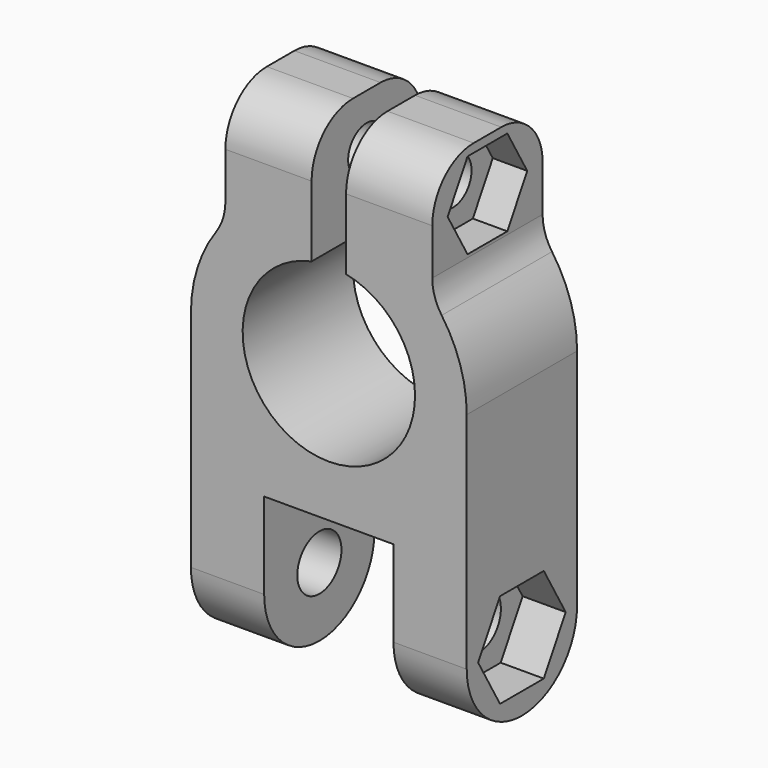
from build123d import *

# Parameters (mm, degrees)
F1_DEPTH = 4
F2_R     = 1.35
F3_DEPTH = 14.001
F4_DEPTH = 2
F5_R     = 1.6
F6_DEPTH = 25
F7_DEPTH = 2.5
F8_SIZE  = 1.35
F9_R     = 3
F10_R    = 3.99999
F11_SIZE = 1.55


# Not quite as in the source:
# - a fillet or chamfer is up to 0.001 mm smaller than in the source, because OpenCascade refuses the exact size
# - a feature names something its author has since deleted; it is built from what else it names


with BuildPart() as f1:
    # F0 (on Front) → F1 (new body, symmetric)
    with BuildSketch(Plane.XZ):
        with BuildLine():
            ThreePointArc((1, 4.8989794856), (0, -5), (-1, 4.8989794856))
            Line((-1, 4.8989794856), (-1, 12))
            Line((-1, 12), (-6, 12))
            Line((-6, 12), (-6, 5.2915026221))
            ThreePointArc((-6, 5.2915026221), (-7.4833147735, 2.8284271247), (-8, 0))
            Line((-8, 0), (-8, -17))
            Line((-8, -17), (-3.75, -17))
            Line((-3.75, -17), (-3.75, -8))
            Line((-3.75, -8), (3.75, -8))
            Line((3.75, -8), (3.75, -17))
            Line((3.75, -17), (8, -17))
            Line((8, -17), (8, 0))
            ThreePointArc((8, 0), (7.4833147735, 2.8284271247), (6, 5.2915026221))
            Line((6, 5.2915026221), (6, 12))
            Line((6, 12), (1, 12))
            Line((1, 12), (1, 4.8989794856))
        make_face()
    extrude(amount=F1_DEPTH, both=True)

    # F2 (on face) → F3 (cut, through all)
    with BuildSketch(Plane.YZ.offset(6)):
        with Locations((0, 9)):
            Circle(F2_R)
    extrude(amount=-F3_DEPTH, mode=Mode.SUBTRACT)

    # F2 (on face) → F4 (cut)
    with BuildSketch(Plane.YZ.offset(6)):
        Polygon((2.8867513459, 9), (1.443375673, 11.5), (-1.443375673, 11.5), (-2.8867513459, 9), (-1.443375673, 6.5), (1.443375673, 6.5), align=None)
        with Locations((0, 9)):
            Circle(F2_R, mode=Mode.SUBTRACT)
    extrude(amount=-F4_DEPTH, mode=Mode.SUBTRACT)

    # F5 (on face) → F6 (cut)
    with BuildSketch(Plane.YZ.offset(8)):
        with Locations((0, -13)):
            Circle(F5_R)
    extrude(amount=-F6_DEPTH, mode=Mode.SUBTRACT)

    # F5 (on face) → F7 (cut)
    with BuildSketch(Plane.YZ.offset(8)):
        Polygon((1.5877132403, -10.25), (-1.5877132403, -10.25), (-3.1754264805, -13), (-1.5877132403, -15.75), (1.5877132403, -15.75), (3.1754264805, -13), align=None)
        with Locations((0, -13)):
            Circle(F5_R, mode=Mode.SUBTRACT)
    extrude(amount=-F7_DEPTH, mode=Mode.SUBTRACT)

    # F8
    f8_edges = [f1.edges().sort_by_distance(p)[0] for p in [
        (-6, -1.35, 9),
    ]]
    chamfer(f8_edges, length=F8_SIZE)

    # F9
    f9_edges = [f1.edges().sort_by_distance(p)[0] for p in [
        (-3.5, -4, 12),
        (3.5, -4, 12),
        (3.5, 4, 12),
        (-3.5, 4, 12),
        (6, 0, 5.291503),
        (-6, 0, 5.291503),
    ]]
    fillet(f9_edges, radius=F9_R)

    # F10 (radius 4 in the source; OpenCascade refuses exactly that, so slightly less here)
    f10_edges = [f1.edges().sort_by_distance(p)[0] for p in [
        (5.875, -4, -17),
        (-5.875, -4, -17),
        (-5.875, 4, -17),
        (5.875, 4, -17),
    ]]
    fillet(f10_edges, radius=F10_R)

    # F11
    f11_edges = [f1.edges().sort_by_distance(p)[0] for p in [
        (-8, -1.6, -13),
    ]]
    chamfer(f11_edges, length=F11_SIZE)


solid = f1.part
